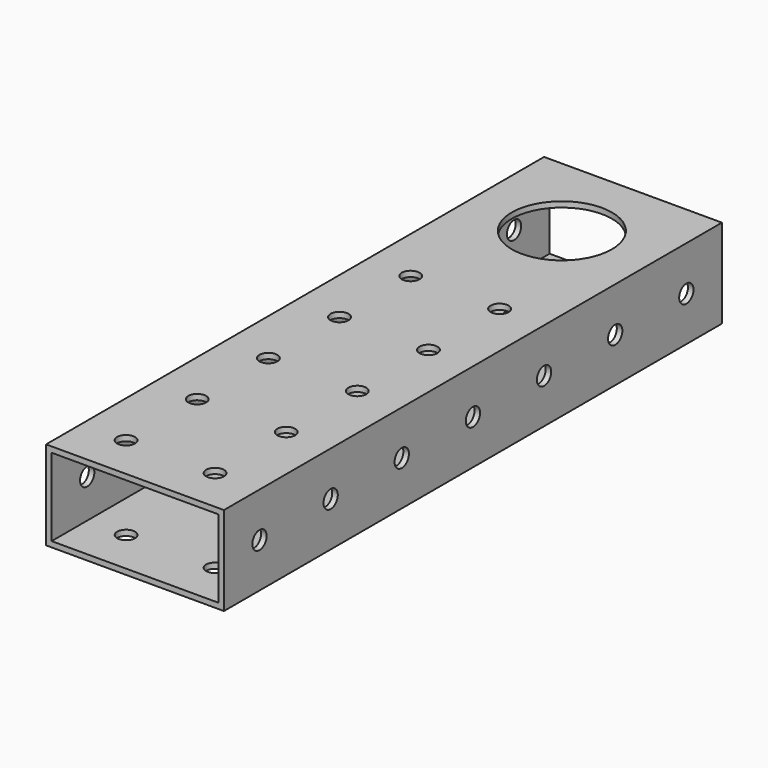
from build123d import *

# Parameters (mm, degrees)
F0_W     = 50.8
F0_H     = 25.4
F1_DEPTH = 177.8
F3_W     = 47.625
F3_H     = 22.225
F4_DEPTH = 203.2
F2_R     = 2.5527
F5_DEPTH = 76.2
F6_R     = 2.5527
F7_DEPTH = 50.8
F6_R_2   = 14.2875
F8_DEPTH = 50.8


# Not quite as in the source:
# - a feature names something its author has since deleted; it is built from what else it names


with BuildPart() as f1:
    # F0 (on Front) → F1 (new body)
    with BuildSketch(Plane.XZ):
        Rectangle(F0_W, F0_H)
    extrude(amount=F1_DEPTH)

    # F3 (on face) → F4 (cut)
    with BuildSketch(Plane.XZ.offset(177.8)):
        Rectangle(F3_W, F3_H)
    extrude(amount=-F4_DEPTH, mode=Mode.SUBTRACT)

    # F2 (on face) → F5 (cut)
    with BuildSketch(Plane.YZ.offset(25.4)):
        with Locations((-165.1, 0)):
            Circle(F2_R)
        with Locations((-139.7, 0)):
            Circle(F2_R)
        with Locations((-114.3, 0)):
            Circle(F2_R)
        with Locations((-88.9, 0)):
            Circle(F2_R)
        with Locations((-63.5, 0)):
            Circle(F2_R)
        with Locations((-38.1, 0)):
            Circle(F2_R)
        with Locations((-12.7, 0)):
            Circle(F2_R)
        with Locations((12.7, 0)):
            Circle(F2_R)
    extrude(amount=-F5_DEPTH, mode=Mode.SUBTRACT)

    # F6 (on face) → F7 (cut)
    with BuildSketch(Plane(origin=(0, 0, -12.7), x_dir=(1, 0, 0), z_dir=(0, 0, -1))):
        with Locations((-12.7, 165.1)):
            Circle(F6_R)
        with Locations((-12.7, 139.7)):
            Circle(F6_R)
        with Locations((-12.7, 114.3)):
            Circle(F6_R)
        with Locations((-12.7, 88.9)):
            Circle(F6_R)
        with Locations((-12.7, 63.5)):
            Circle(F6_R)
        with Locations((12.7, 63.5)):
            Circle(F6_R)
        with Locations((12.7, 88.9)):
            Circle(F6_R)
        with Locations((12.7, 114.3)):
            Circle(F6_R)
        with Locations((12.7, 139.7)):
            Circle(F6_R)
        with Locations((12.7, 165.1)):
            Circle(F6_R)
    extrude(amount=-F7_DEPTH, mode=Mode.SUBTRACT)

    # F6 (on face) → F8 (cut)
    with BuildSketch(Plane(origin=(0, 0, -12.7), x_dir=(1, 0, 0), z_dir=(0, 0, -1))):
        with Locations((0, 25.4)):
            Circle(F6_R_2)
    extrude(amount=-F8_DEPTH, mode=Mode.SUBTRACT)


solid = f1.part
